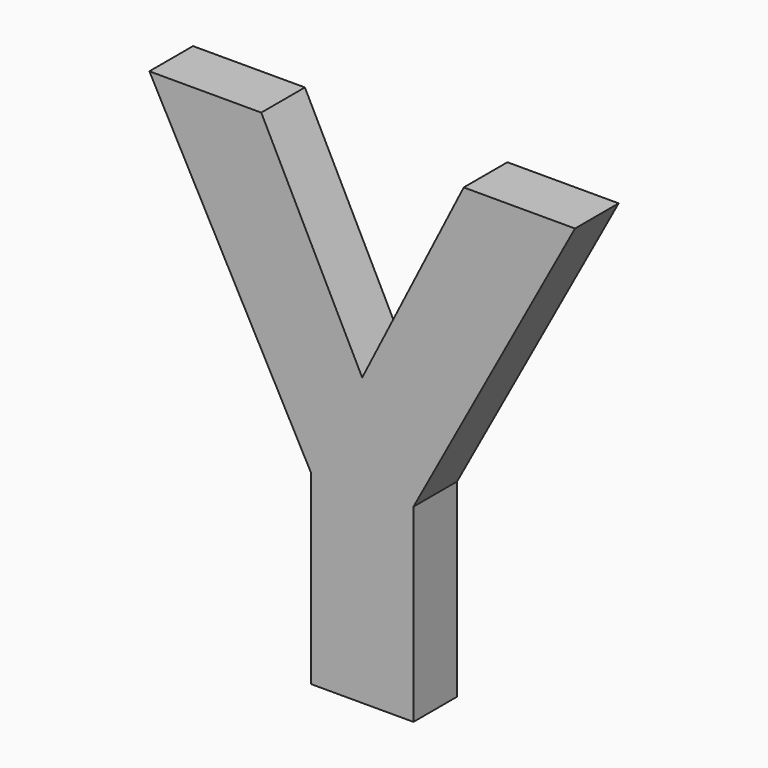
from build123d import *

# Parameters (mm, degrees)
F0_TEXT_SIZE = 62.5
F1_DEPTH     = 5


# Not quite as in the source:
# - Text() gives the source's letters only with a copy of the font that has no kerning and outlines rounded to 1/6400 em; it was checked with that copy


with BuildPart() as f1:
    # F0 (on Front) → F1 (new body)
    with BuildSketch(Plane.XZ):
        with Locations((-72.2301180681, 25.6960258421)):
            Text('Y', F0_TEXT_SIZE, font='Open Sans', font_style=FontStyle.BOLD, text_align=(TextAlign.LEFT, TextAlign.BOTTOM))
    extrude(amount=F1_DEPTH)


solid = f1.part
